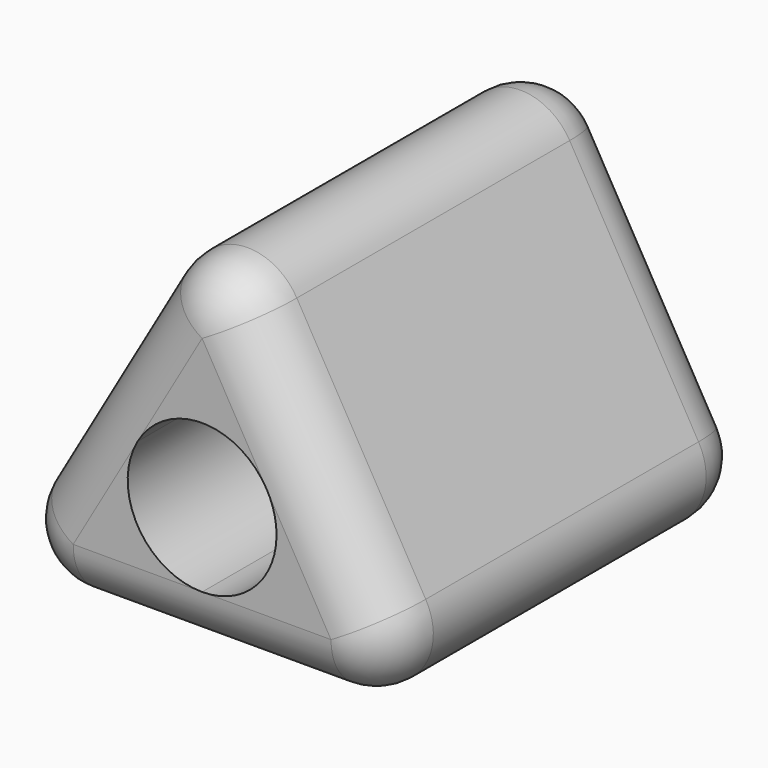
from build123d import *

# Parameters (mm, degrees)
F1_DEPTH      = 50.8
F2_R          = 6.35
F4_DEPTH      = 68.834
F4_DEPTH_BACK = 105


# Not quite as in the source:
# - an extrude ends at something that could not be found from the text; its depth is read off the source's solid


with BuildPart() as f1:
    # F0 (on Front) → F1 (new body)
    with BuildSketch(Plane.XZ):
        Polygon((-25.4, 0), (0, 0), (25.4, 0), (0, 43.9940905122), align=None)
    extrude(amount=F1_DEPTH)

    # F2
    f2_edges = [f1.edges().sort_by_distance(p)[0] for p in [
        (0, -25.4, 43.994091),
        (12.7, -50.8, 21.997045),
        (-12.7, -50.8, 21.997045),
        (0, -50.8, 0),
        (25.4, -25.4, 0),
        (12.7, 0, 21.997045),
        (0, 0, 0),
        (-12.7, 0, 21.997045),
        (-25.4, -25.4, 0),
    ]]
    fillet(f2_edges, radius=F2_R)

    # F3 (on face) → F4 (cut, two sides)
    with BuildSketch(Plane.XZ.offset(50.8)) as f4_sk:
        with BuildLine():
            ThreePointArc((0, 6.35), (5.8793785172, 8.7853183202), (8.3146968374, 14.6646968374))
            ThreePointArc((8.3146968374, 14.6646968374), (8.0313803879, 16.8166988268), (7.200738589, 18.822045424))
            ThreePointArc((7.200738589, 18.822045424), (-9.37e-08, 22.9793936748), (-7.2007386828, 18.8220452616))
            ThreePointArc((-7.2007386828, 18.8220452616), (-7.2007386876, 10.5073484215), (0, 6.35))
        make_face()
    extrude(amount=-F4_DEPTH, mode=Mode.SUBTRACT)
    extrude(f4_sk.sketch, amount=F4_DEPTH_BACK, mode=Mode.SUBTRACT)


solid = f1.part
